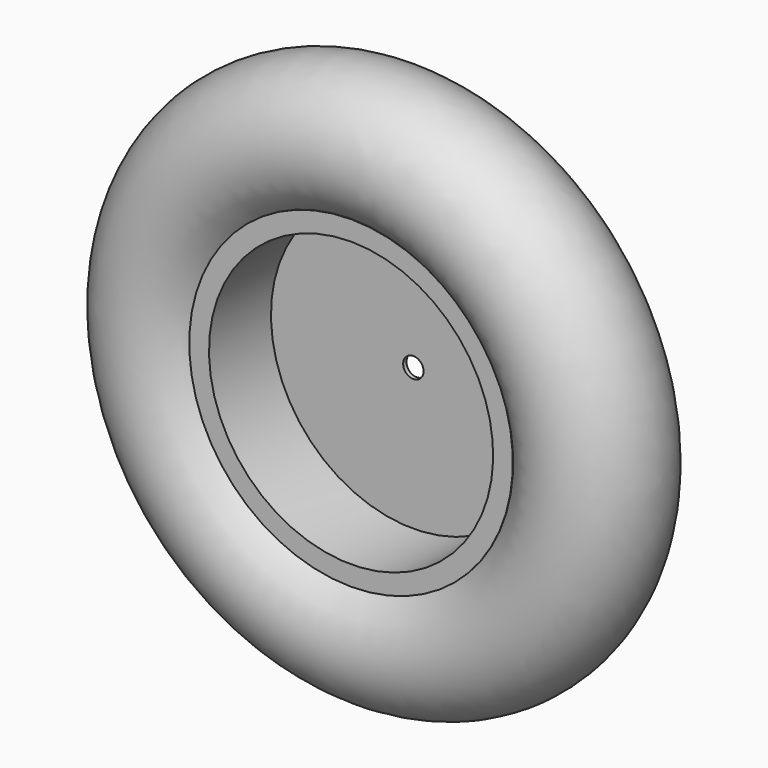
from build123d import *

# Parameters (mm, degrees)
F0_R     = 88.9
F0_R_2   = 6.35
F1_DEPTH = 2.54


with BuildPart() as f1:
    # F0 (on Front) → F1 (new body)
    with BuildSketch(Plane.XZ):
        with Locations((-0.2168306673, 0.1073895255)):
            Circle(F0_R)
        Circle(F0_R_2, mode=Mode.SUBTRACT)
    extrude(amount=F1_DEPTH)

    # F2 (on Right) → F3 (revolve)
    with BuildSketch(Plane.YZ):
        with BuildLine():
            Line((-50.5609217677, 100.939810276), (-50.8, 100.939810276))
            Line((-50.8, 100.939810276), (-50.8, 88.648326695))
            Line((-50.8, 88.648326695), (0, 88.648326695))
            Line((0, 88.648326695), (0, 100.78047497))
            ThreePointArc((0, 100.78047497), (-25.3081661852, 92.0685846893), (-50.5609217677, 100.939810276))
        make_face()
        with BuildLine():
            ThreePointArc((15.5636772252, 132.8118294477), (-42.8703444402, 169.5143096026), (-50.5609217677, 100.939810276))
            Line((-50.5609217677, 100.939810276), (0, 100.939810276))
            Line((0, 100.939810276), (0, 100.78047497))
            ThreePointArc((0, 100.78047497), (11.4667790995, 115.0056808015), (15.5636772252, 132.8118294477))
        make_face()
        with BuildLine():
            Line((0, 100.939810276), (-50.5609217677, 100.939810276))
            ThreePointArc((-50.5609217677, 100.939810276), (-25.3081661852, 92.0685846893), (0, 100.78047497))
            Line((0, 100.78047497), (0, 100.939810276))
        make_face()
    revolve(axis=Axis((-0.2168306673, -2.54, 0.1073895255), (0, -1, 0)))


solid = f1.part
